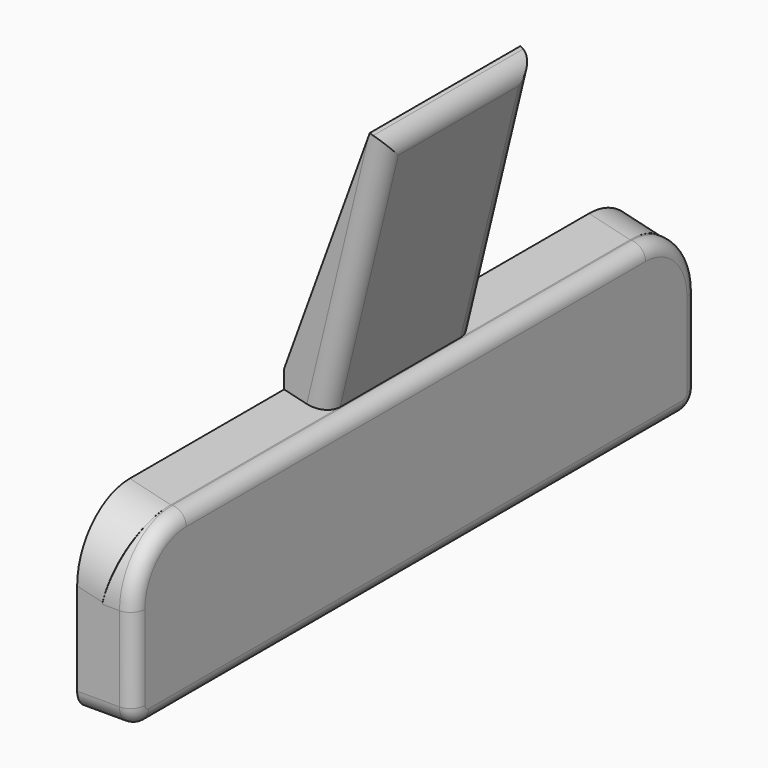
from build123d import *

# Parameters (mm, degrees)
F1_DEPTH     = 6
F2_R         = 1.5
F4_DEPTH     = 75
F6_DEPTH     = 10.8061096393
F7_T1_DEPTH  = 28.1827713518
F7_T6_DEPTH  = 32.9363939608
F7_T11_DEPTH = 32.9363939608
F8_W         = 10
F8_H         = 10
F9_DEPTH     = 2
F10_R        = 2.4
F11_DEPTH    = 2


# Not quite as in the source:
# - a fillet or chamfer that OpenCascade refuses, or shapes differently, is made with other operations: its cross-section is extruded or revolved along the edge and cut away or added


with BuildPart() as f1:
    # F0 (on Right) → F1 (new body)
    with BuildSketch(Plane.YZ):
        with BuildLine():
            Line((-35.5, 0), (35.5, 0))
            ThreePointArc((35.5, 0), (36.9142135624, 0.5857864376), (37.5, 2))
            Line((37.5, 2), (37.5, 11))
            ThreePointArc((37.5, 11), (35.4497474683, 15.9497474683), (30.5, 18))
            Line((30.5, 18), (-30.5, 18))
            ThreePointArc((-30.5, 18), (-35.4497474683, 15.9497474683), (-37.5, 11))
            Line((-37.5, 11), (-37.5, 2))
            ThreePointArc((-37.5, 2), (-36.9142135624, 0.5857864376), (-35.5, 0))
        make_face()
    extrude(amount=F1_DEPTH)

    # F2
    f2_edges = [f1.edges().sort_by_distance(p)[0] for p in [
        (6, 37.5, 6.5),
        (6, 0, 0),
        (6, 36.914214, 0.585786),
        (6, 35.449747, 15.949747),
        (6, 0, 18),
        (6, -35.449747, 15.949747),
        (6, -37.5, 6.5),
        (6, -36.914214, 0.585786),
    ]]
    fillet(f2_edges, radius=F2_R)

    # F3 (on face) → F4 (join, through all)
    with BuildSketch(Plane(origin=(0, 37.5, 0), x_dir=(-1, 0, 0), z_dir=(0, 1, 0))):
        Polygon((0, 21), (-9.0992558567, 46), (-10.9118714307, 45.1547634765), (-2.6582042845, 11), (0, 11), align=None)
    extrude(amount=-F4_DEPTH)

    # F5 (on face) → F6 (cut, through all)
    with BuildSketch(Plane(origin=(0, 0, 0), x_dir=(0, 1, 0), z_dir=(0.9720210674, 0, -0.2348936878))):
        with BuildLine():
            ThreePointArc((30.5, 18.5181171521), (35.4497474683, 16.4678646204), (37.5, 11.5181171521))
            Line((37.5, 11.5181171521), (37.5, 48.565749079))
            Line((37.5, 48.565749079), (10, 48.565749079))
            Line((10, 48.565749079), (10, 18.5181171521))
            Line((10, 18.5181171521), (30.5, 18.5181171521))
        make_face()
        with BuildLine():
            Line((-10, 48.565749079), (-37.5, 48.565749079))
            Line((-37.5, 48.565749079), (-37.5, 11.5181171521))
            ThreePointArc((-37.5, 11.5181171521), (-35.4497474683, 16.4678646204), (-30.5, 18.5181171521))
            Line((-30.5, 18.5181171521), (-10, 18.5181171521))
            Line((-10, 18.5181171521), (-10, 48.565749079))
        make_face()
    extrude(amount=-F6_DEPTH, mode=Mode.SUBTRACT)

    # F7: fillet of radius 2 on 3 edges, made by hand

    # F7_s2 → F7_t1 (cut)
    with BuildSketch(Plane.XZ.offset(-14.0913856759)):
        with BuildLine():
            ThreePointArc((10.5274551629, 43.5639982478), (10.3854562197, 44.9013340863), (9.4286495516, 45.8464011975))
            Line((9.4286495516, 45.8464011975), (10.9118714307, 45.1547634765))
            Line((10.9118714307, 45.1547634765), (10.5274551629, 43.5639982478))
        make_face()
    extrude(amount=F7_T1_DEPTH, mode=Mode.SUBTRACT)


with BuildPart() as f7_tool4:
    # F7_s5 → F7_t6 (new body)
    with BuildSketch(Plane(origin=(12.0863398698, 0, 50.0148688134), x_dir=(0, 1, 0), z_dir=(-0.2348936878, 0, -0.9720210674))):
        with BuildLine():
            ThreePointArc((10, -2), (9.4142135624, -0.5857864376), (8, 0))
            Line((8, 0), (10, 0))
            Line((10, 0), (10, -2))
        make_face()
    extrude(amount=F7_T6_DEPTH)

    split(bisect_by=Plane.XY.offset(18), keep=Keep.TOP)


with BuildPart() as f1_1:
    add(f1.part)

    # F7_t3: cut F7_tool4
    add(f7_tool4.part, mode=Mode.SUBTRACT)


with BuildPart() as f7_tool9:
    # F7_s10 → F7_t11 (new body)
    with BuildSketch(Plane(origin=(4.3497888292, 0, 18), x_dir=(0, 1, 0), z_dir=(0.2348936878, 0, 0.9720210674))):
        with BuildLine():
            ThreePointArc((-10, 2), (-9.4142135624, 0.5857864376), (-8, 0))
            Line((-8, 0), (-10, 0))
            Line((-10, 0), (-10, 2))
        make_face()
    extrude(amount=F7_T11_DEPTH)

    split(bisect_by=Plane.XY.offset(18), keep=Keep.TOP)


with BuildPart() as f1_2:
    add(f1_1.part)

    # F7_t8: cut F7_tool9
    add(f7_tool9.part, mode=Mode.SUBTRACT)

    # F8 (on face) → F9 (cut)
    with BuildSketch(Plane(origin=(-6.7492699017, 0, 2.4565333473), x_dir=(0, -1, 0), z_dir=(-0.9396926208, 0, 0.3420201433))):
        with Locations((0, 29.7335450365)):
            Rectangle(F8_W, F8_H)
    extrude(amount=-F9_DEPTH, mode=Mode.SUBTRACT)

    # F10 (on face) → F11 (join)
    with BuildSketch(Plane(origin=(-4.8698846601, 0, 1.7724930606), x_dir=(0, -1, 0), z_dir=(-0.9396926208, 0, 0.3420201433))):
        with Locations((0, 29.7335450365)):
            Circle(F10_R)
    extrude(amount=F11_DEPTH)


solid = f1_2.part
